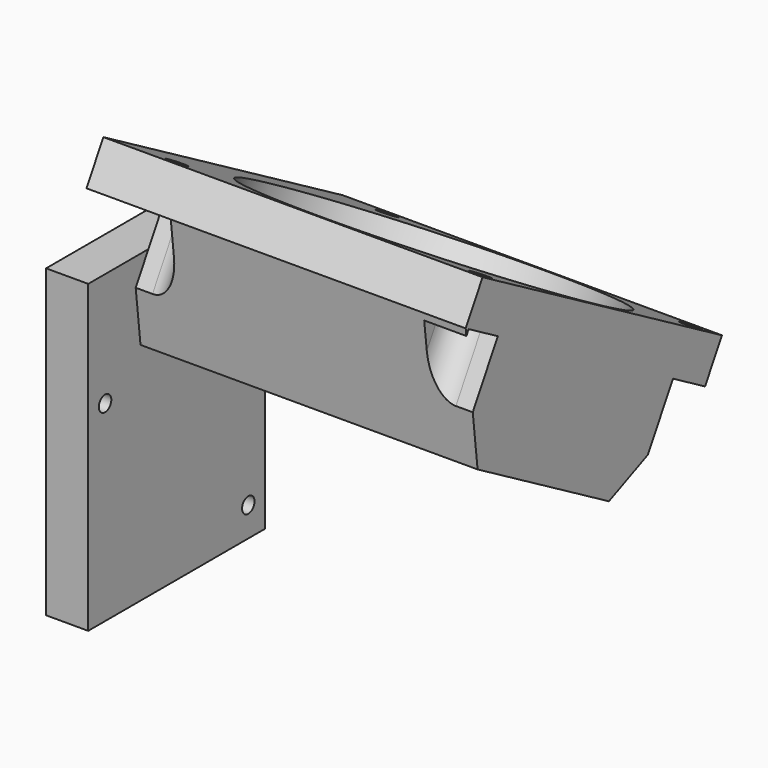
from build123d import *

# Parameters (mm, degrees)
F0_W      = 52.5
F0_H      = 72.5
F0_R      = 1.85
F1_DEPTH  = 10
F3_W      = 90
F3_H      = 10
F4_DEPTH  = 41
F5_R      = 2.25
F5_R_2    = 39
F7_DEPTH  = 89.0378417744
F9_W      = 80
F9_H      = 82
F8_W      = 80
F8_H      = 45
F11_R     = 39
F12_R     = 20
F15_DEPTH = 25


with BuildPart() as f1:
    # F0 (on Right) → F1 (new body)
    with BuildSketch(Plane.YZ):
        with Locations((0, 36.25)):
            Rectangle(F0_W, F0_H)
        with Locations((21.25, 7)):
            Circle(F0_R, mode=Mode.SUBTRACT)
        with Locations((-21.25, 45.5)):
            Circle(F0_R, mode=Mode.SUBTRACT)
    extrude(amount=F1_DEPTH)

    # F3 (on face) → F4 (join, symmetric)
    with BuildSketch(Plane(origin=(0, -11.7059208872, 6.7584165753), x_dir=(-1, 0, 0), z_dir=(0, 0.8660254038, -0.5))):
        with Locations((-45, 70.9118417744)):
            Rectangle(F3_W, F3_H)
    extrude(amount=F4_DEPTH, both=True)

    # F5 (on face) → F7 (cut, through all)
    with BuildSketch(Plane(origin=(0, 37.9559208872, 65.7415834247), x_dir=(1, 0, 0), z_dir=(0, 0.5, 0.8660254038))):
        with Locations((14, -49.5168331507)):
            Circle(F5_R)
        with Locations((86, -49.5168331507)):
            Circle(F5_R)
        with Locations((86, 22.4831668493)):
            Circle(F5_R)
        with Locations((14, 22.4831668493)):
            Circle(F5_R)
        with Locations((50, -13.5168331507)):
            Circle(F5_R_2)
    extrude(amount=-F7_DEPTH, mode=Mode.SUBTRACT)

    # F9 (on face) → F10 section 0
    with BuildSketch(Plane(origin=(0, 32.9559208872, 57.0813293868), x_dir=(1, 0, 0), z_dir=(0, -0.5, -0.8660254038))):
        with Locations((50, 13.5168331507)):
            Rectangle(F9_W, F9_H)
    # F8 (on offset) → F10 section 1
    with BuildSketch(Plane(origin=(0, 20.4559208872, 35.4306942922), x_dir=(1, 0, 0), z_dir=(0, -0.5, -0.8660254038))):
        with Locations((50, 13.5168331507)):
            Rectangle(F8_W, F8_H)
    loft()

    # F11 (on face) → F13 section 0
    with BuildSketch(Plane(origin=(0, 32.9559208872, 57.0813293868), x_dir=(1, 0, 0), z_dir=(0, -0.5, -0.8660254038))):
        with Locations((50, 13.5168331507)):
            Circle(F11_R)
    # F12 (on face) → F13 section 1
    with BuildSketch(Plane(origin=(0, 20.4559208872, 35.4306942922), x_dir=(1, 0, 0), z_dir=(0, -0.5, -0.8660254038))):
        with Locations((50, 13.5168331507)):
            Circle(F12_R)
    loft(mode=Mode.SUBTRACT)

    # F14 (on face) → F15 (cut, through all)
    with BuildSketch(Plane(origin=(0, 32.9559208872, 57.0813293868), x_dir=(1, 0, 0), z_dir=(0, -0.5, -0.8660254038))):
        with BuildLine():
            Line((10, 43.5168331507), (14, 43.5168331507))
            ThreePointArc((14, 43.5168331507), (18.2426406871, 45.2741924635), (20, 49.5168331507))
            Line((20, 49.5168331507), (20, 54.5168331507))
            Line((20, 54.5168331507), (10, 54.5168331507))
            Line((10, 54.5168331507), (10, 43.5168331507))
        make_face()
        with BuildLine():
            Line((9, -26.4831668493), (20, -26.4831668493))
            Line((20, -26.4831668493), (20, -22.4831668493))
            ThreePointArc((20, -22.4831668493), (18.2426406871, -18.2405261622), (14, -16.4831668493))
            Line((14, -16.4831668493), (9, -16.4831668493))
            Line((9, -16.4831668493), (9, -26.4831668493))
        make_face()
        with BuildLine():
            Line((90, -27.4831668493), (90, -16.4831668493))
            Line((90, -16.4831668493), (86, -16.4831668493))
            ThreePointArc((86, -16.4831668493), (81.7573593129, -18.2405261622), (80, -22.4831668493))
            Line((80, -22.4831668493), (80, -27.4831668493))
            Line((80, -27.4831668493), (90, -27.4831668493))
        make_face()
        with BuildLine():
            Line((91, 53.5168331507), (80, 53.5168331507))
            Line((80, 53.5168331507), (80, 49.5168331507))
            ThreePointArc((80, 49.5168331507), (81.7573593129, 45.2741924635), (86, 43.5168331507))
            Line((86, 43.5168331507), (91, 43.5168331507))
            Line((91, 43.5168331507), (91, 53.5168331507))
        make_face()
    extrude(amount=F15_DEPTH, mode=Mode.SUBTRACT)


solid = f1.part
